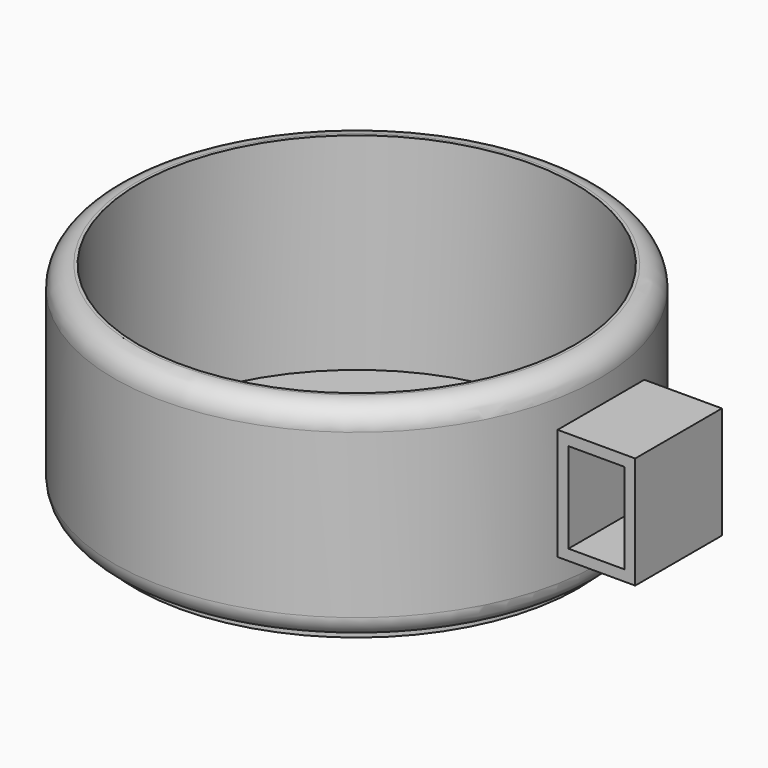
from build123d import *

# Parameters (mm, degrees)
F0_R        = 56.8614302175
F0_R_2      = 51.0824903335
F1_DEPTH    = 48.3736
F2_R        = 51.8810866732
F3_DEPTH    = 1.62169
F4_W        = 18.1773193181
F4_H        = 26.2230178341
F5_DEPTH    = 12.7
F6_T        = -2.54
F7_R        = 5.08
F8_S5_R     = 51.8810866732
F8_T6_DEPTH = 89


# Not quite as in the source:
# - a fillet or chamfer that OpenCascade refuses, or shapes differently, is made with other operations: its cross-section is extruded or revolved along the edge and cut away or added


with BuildPart() as f1:
    # F0 (on Top) → F1 (new body)
    with BuildSketch(Plane.XY):
        Circle(F0_R)
        Circle(F0_R_2, mode=Mode.SUBTRACT)
    extrude(amount=F1_DEPTH)

    # F2 (on Top) → F3 (join)
    with BuildSketch(Plane.XY):
        Circle(F2_R)
    extrude(amount=-F3_DEPTH)

    # F7
    f7_edges = [f1.edges().sort_by_distance(p)[0] for p in [
        (-56.86143, 0, 48.3736),
    ]]
    fillet(f7_edges, radius=F7_R)

    # F8: fillet of radius 5.08 on 1 edges, made by hand


with BuildPart() as f5:
    # F4 (on Front) → F5 (new body, symmetric)
    with BuildSketch(Plane.XZ):
        with Locations((66.3025137037, 24.8820674606)):
            Rectangle(F4_W, F4_H)
    extrude(amount=F5_DEPTH, both=True)

    # F6
    f6_openings = [f5.faces().sort_by_distance(p)[0] for p in [
        (66.302514, -12.7, 24.882067),
        (66.302514, 12.7, 24.882067),
    ]]
    offset(amount=F6_T, openings=f6_openings)


with BuildPart() as f8_tool2:
    # F8_s3 → F8_t4 (revolve)
    with BuildSketch(Plane.XZ):
        with BuildLine():
            ThreePointArc((56.8614302175, 5.08), (55.3735326659, 1.4878975516), (51.7814302175, 0))
            Line((51.7814302175, 0), (56.8614302175, 0))
            Line((56.8614302175, 0), (56.8614302175, 5.08))
        make_face()
    revolve(axis=Axis((0, 0, 0), (0, 0, 1)))

    # F8_s5 → F8_t6 (cut, symmetric)
    with BuildSketch(Plane.XY.offset(2.5)):
        Circle(F8_S5_R)
    extrude(amount=F8_T6_DEPTH, both=True, mode=Mode.SUBTRACT)


with BuildPart() as f1_1:
    add(f1.part)

    # F8_t1: cut F8_tool2
    add(f8_tool2.part, mode=Mode.SUBTRACT)


solid = Compound([f5.part, f1_1.part])
